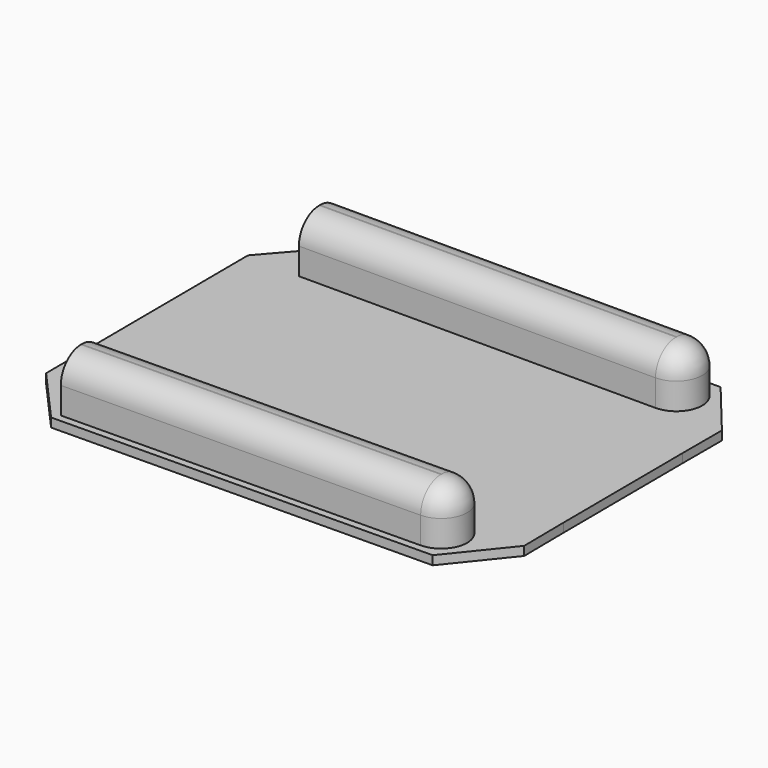
from build123d import *

# Parameters (mm, degrees)
F2_DEPTH = 25.4
F3_W     = 1016
F3_H     = 147.955
F4_DEPTH = 147.955
F5_DEPTH = 133.5532
F6_R     = 72.39
F7_R     = 72.39


# Not quite as in the source:
# - a feature names something its author has since deleted; it is built from what else it names


with BuildPart() as f2:
    # F1 (on face) → F2 (new body)
    with BuildSketch(Plane.XY):
        Polygon((319.0343479268, 457.2), (236.3300025423, 362.0783686638), (240.3907269744, -362.0321180929), (325.0280779844, -457.2), (1501.5633212704, -457.2), (1590.3160302528, -346.8912047778), (1588.7331709988, -205.7675014721), (1587.5366926193, 7.5891437009), (1586.3402142398, 220.9457888739), (1586.3402142398, 362.0783686638), (1508.033296253, 457.2), align=None)
        Polygon((376.3225418129, 523.0894817851), (319.0343479268, 457.2), (1508.033296253, 457.2), (1453.79114151, 523.0894817851), align=None)
        Polygon((1501.5633212704, -457.2), (325.0280779844, -457.2), (382.1802665493, -521.4630312406), (1459.5810992365, -509.3787828947), align=None)
    extrude(amount=F2_DEPTH)

    # F3 (on face) → F4 (join)
    with BuildSketch(Plane.XY.offset(25.4)):
        with Locations((895.4748051167, 428.2288251305)):
            Rectangle(F3_W, F3_H)
        with BuildLine():
            Line((1403.4748051167, 502.2063251305), (1403.4748051167, 354.2513251305))
            ThreePointArc((1403.4748051167, 354.2513251305), (1477.4523051167, 428.2288251305), (1403.4748051167, 502.2063251305))
        make_face()
        Polygon((391.4505850052, -352.5514191944), (393.1150321411, -500.4970566453), (1409.0507399579, -489.0673767425), (1407.3862928221, -341.1217392917), align=None)
        with BuildLine():
            Line((1407.3862928221, -341.1217392917), (1409.0507399579, -489.0673767425))
            ThreePointArc((1409.0507399579, -489.0673767425), (1482.1913351154, -414.2623344491), (1407.3862928221, -341.1217392917))
        make_face()
    extrude(amount=F4_DEPTH)

    # F3 (on face) → F5 (join)
    with BuildSketch(Plane.XY.offset(25.4)):
        with Locations((895.4748051167, 428.2288251305)):
            Rectangle(F3_W, F3_H)
        with BuildLine():
            Line((1403.4748051167, 502.2063251305), (1403.4748051167, 354.2513251305))
            ThreePointArc((1403.4748051167, 354.2513251305), (1477.4523051167, 428.2288251305), (1403.4748051167, 502.2063251305))
        make_face()
        Polygon((391.4505850052, -352.5514191944), (393.1150321411, -500.4970566453), (1409.0507399579, -489.0673767425), (1407.3862928221, -341.1217392917), align=None)
        with BuildLine():
            Line((1407.3862928221, -341.1217392917), (1409.0507399579, -489.0673767425))
            ThreePointArc((1409.0507399579, -489.0673767425), (1482.1913351154, -414.2623344491), (1407.3862928221, -341.1217392917))
        make_face()
    extrude(amount=F5_DEPTH)

    # F6
    f6_edges = [f2.edges().sort_by_distance(p)[0] for p in [
        (895.474805, 502.206325, 173.355),
        (1477.452305, 428.228825, 173.355),
        (895.474805, 354.251325, 173.355),
    ]]
    fillet(f6_edges, radius=F6_R)

    # F7
    f7_edges = [f2.edges().sort_by_distance(p)[0] for p in [
        (899.418439, -346.836579, 173.355),
        (1482.191335, -414.262334, 173.355),
        (901.082886, -494.782217, 173.355),
    ]]
    fillet(f7_edges, radius=F7_R)


solid = f2.part
